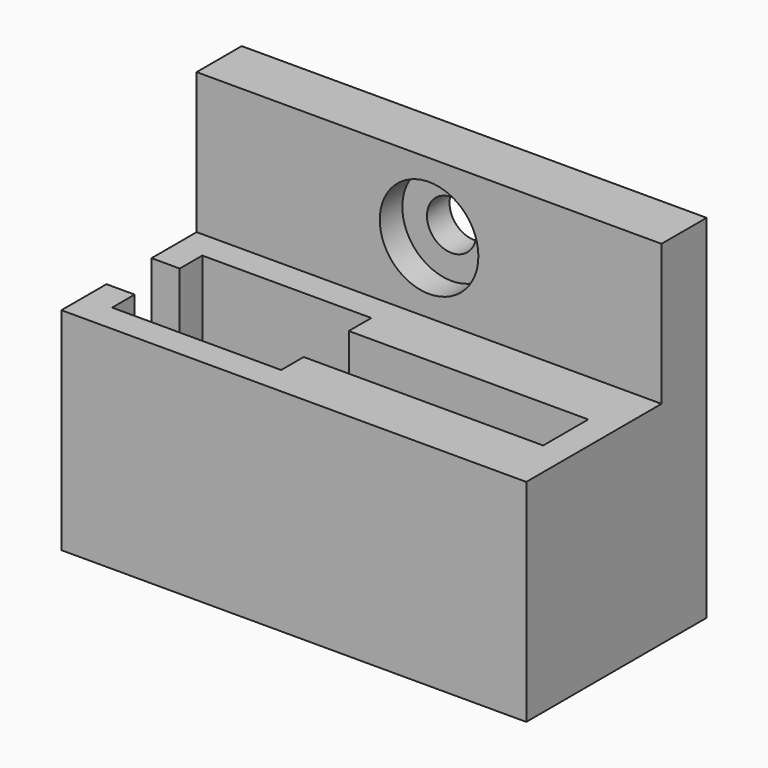
from build123d import *

# Parameters (mm, degrees)
F0_W     = 33
F0_H     = 4
F1_DEPTH = 25
F0_W_2   = 12
F0_H_2   = 2
F2_DEPTH = 3
F3_DEPTH = 15
F4_R     = 1.75
F5_DEPTH = 25
F4_R_2   = 3.5
F6_DEPTH = 2


with BuildPart() as f1:
    # F0 (on Top) → F1 (new body)
    with BuildSketch(Plane.XY):
        with Locations((16.5, 14)):
            Rectangle(F0_W, F0_H)
    extrude(amount=F1_DEPTH)

    # F0 (on Top) → F3 (join)
    with BuildSketch(Plane.XY):
        Polygon((0, 4), (0, 0), (33, 0), (33, 12), (0, 12), (0, 8), (2, 8), (2, 10), (14, 10), (14, 8), (31, 8), (31, 4), (14, 4), (14, 2), (2, 2), (2, 4), align=None)
    extrude(amount=F3_DEPTH)

    # F4 (on face) → F5 (cut)
    with BuildSketch(Plane.XZ.offset(-12)):
        with Locations((16.5, 20)):
            Circle(F4_R)
    extrude(amount=-F5_DEPTH, mode=Mode.SUBTRACT)

    # F4 (on face) → F6 (cut)
    with BuildSketch(Plane.XZ.offset(-12)):
        with Locations((16.5, 20)):
            Circle(F4_R_2)
        with Locations((16.5, 20)):
            Circle(F4_R, mode=Mode.SUBTRACT)
    extrude(amount=-F6_DEPTH, mode=Mode.SUBTRACT)


with BuildPart() as f2:
    # F0 (on Top) → F2 (new body)
    with BuildSketch(Plane.XY):
        with Locations((8, 9)):
            Rectangle(F0_W_2, F0_H_2)
    extrude(amount=F2_DEPTH)


with BuildPart() as f2b:
    # F0 (on Top) → F2, piece 2 (new body)
    with BuildSketch(Plane.XY):
        with Locations((8, 3)):
            Rectangle(F0_W_2, F0_H_2)
    extrude(amount=F2_DEPTH)


solid = Compound([f1.part, f2.part, f2b.part])
